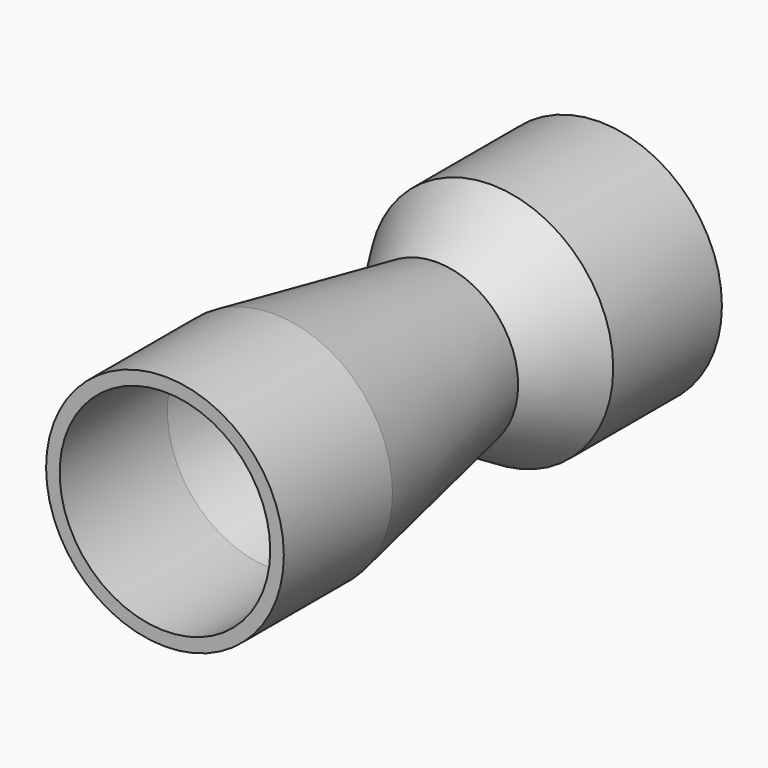
from build123d import *

# Parameters (mm, degrees)
F0_R         = 8.75
F4_R         = 6
F6_DEPTH     = 10
F10_R        = 9
F5_FACE1_R   = 6
F12_DEPTH    = 10
F13_T        = 1
F13_T4_ANGLE = 180.000000001
F13_T6_ANGLE = 180.000000001


# Not quite as in the source:
# - a shell that OpenCascade refuses in one call is made with other operations: the cavity is built on its own and cut out


with BuildPart() as f5:
    # F0 (on Front) → F5 section 0
    with BuildSketch(Plane.XZ):
        Circle(F0_R)
    # F4 (on line) → F5 section 1
    with BuildSketch(Plane(origin=(0, 15, 0), x_dir=(-1, 0, 0), z_dir=(0, 1, 0))):
        Circle(F4_R)
    loft()

    # F6 (add): a face of the model
    f6_faces = [f5.faces().sort_by_distance(p)[0] for p in [
        (0, 0, 0),
    ]]
    extrude(f6_faces, amount=F6_DEPTH)

    # F10 (on line) → F11 section 0
    with BuildSketch(Plane(origin=(0, 20, 0), x_dir=(-1, 0, 0), z_dir=(0, 1, 0))):
        Circle(F10_R)
    # F5_face1 (on face) → F11 section 1
    with BuildSketch(Plane(origin=(0, 15, 0), x_dir=(-1, 0, 0), z_dir=(0, 1, 0))):
        Circle(F5_FACE1_R)
    loft()

    # F12 (add): a face of the model
    f12_faces = [f5.faces().sort_by_distance(p)[0] for p in [
        (0, 20, 0),
    ]]
    extrude(f12_faces, amount=F12_DEPTH)

    # F13: shell of thickness 1, made by hand


with BuildPart() as f13_core1:
    # F13_t2: copy of F5
    add(f5.part)

    # the walls: a layer under each face that stays
    f13_faces = [f13_core1.faces().sort_by_distance(p)[0] for p in [
        (-7.375, 7.5, 0),
        (7.5, 17.5, 0),
        (-8.75, -5, 0),
        (9, 25, 0),
    ]]
    thicken(f13_faces, amount=-F13_T, mode=Mode.SUBTRACT)

    # F13_s3 → F13_t4 (revolve, cut)
    with BuildSketch(Plane.XY):
        Polygon((6.0184109948, 14.9966583211), (5.0163934426, 14.8196721311), (4.9483384219, 15.1908813349), (5.1425070743, 15.5144957554), align=None)
    revolve(axis=Axis((0, 15, 0), (0, -1, 0)), revolution_arc=F13_T4_ANGLE, mode=Mode.SUBTRACT)

    # F13_s5 → F13_t6 (revolve, cut)
    with BuildSketch(Plane.XY):
        Polygon((-6.0184109948, 14.9966583211), (-5.0163934426, 14.8196721311), (-4.9483384219, 15.1908813349), (-5.1425070743, 15.5144957554), align=None)
    revolve(axis=Axis((0, 15, 0), (0, -1, 0)), revolution_arc=F13_T6_ANGLE, mode=Mode.SUBTRACT)


with BuildPart() as f5_1:
    add(f5.part)

    # what is left inside the walls is the cavity
    f13_cavity = [f13_core1.part.solids().sort_by_distance(p)[0] for p in [
        (-6.828962, 4.877481, 0),
    ]]
    add(f13_cavity, mode=Mode.SUBTRACT)


solid = f5_1.part
